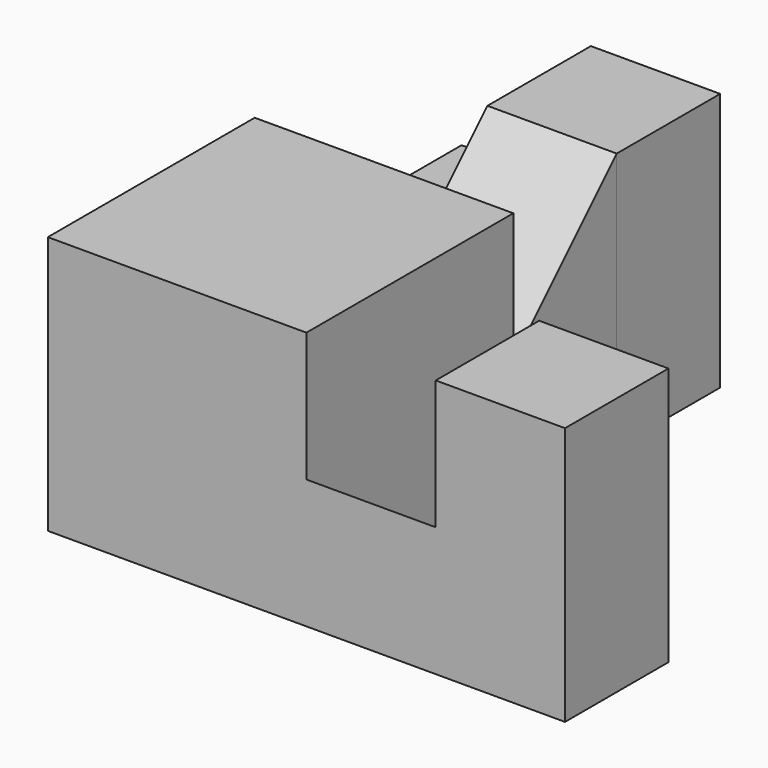
from build123d import *

# Parameters (mm, degrees)
F0_W     = 8
F0_H     = 8
F1_DEPTH = 16
F2_DEPTH = 8
F3_DEPTH = 16
F4_DEPTH = 8
F5_DEPTH = 16
F6_DEPTH = 16
F7_SIZE  = 7.99999
F8_SIZE  = 7.99999


# Not quite as in the source:
# - a fillet or chamfer is up to 0.001 mm smaller than in the source, because OpenCascade refuses the exact size


with BuildPart() as f1:
    # F0 (on Top) → F1 (new body)
    with BuildSketch(Plane.XY):
        with Locations((-2.9367977926, -12)):
            Rectangle(F0_W, F0_H)
    extrude(amount=F1_DEPTH)

    # F0 (on Top) → F2 (join)
    with BuildSketch(Plane.XY):
        with Locations((-10.9367977926, -12)):
            Rectangle(F0_W, F0_H)
    extrude(amount=F2_DEPTH)

    # F0 (on Top) → F3 (join)
    with BuildSketch(Plane.XY):
        Polygon((-22.9367977926, 0), (-30.9367977926, 0), (-30.9367977926, -16), (-14.9367977926, -16), (-14.9367977926, -8), (-14.9367977926, 0), align=None)
    extrude(amount=F3_DEPTH)

    # F0 (on Top) → F4 (join)
    with BuildSketch(Plane.XY):
        Polygon((-22.9367977926, 16), (-30.9367977926, 16), (-30.9367977926, 0), (-22.9367977926, 0), (-22.9367977926, 8), align=None)
    extrude(amount=F4_DEPTH)

    # F0 (on Top) → F5 (join)
    with BuildSketch(Plane.XY):
        with Locations((-18.9367977926, 12)):
            Rectangle(F0_W, F0_H)
    extrude(amount=F5_DEPTH)

    # F7 (size 8 in the source; OpenCascade refuses exactly that, so slightly less here)
    f7_edges = [f1.edges().sort_by_distance(p)[0] for p in [
        (-10.936798, -8, 8),
    ]]
    chamfer(f7_edges, length=F7_SIZE)


with BuildPart() as f6:
    # F0 (on Top) → F6 (new body)
    with BuildSketch(Plane.XY):
        with Locations((-18.9367977926, 4)):
            Rectangle(F0_W, F0_H)
    extrude(amount=F6_DEPTH)

    # F8 (size 8 in the source; OpenCascade refuses exactly that, so slightly less here)
    f8_edges = [f6.edges().sort_by_distance(p)[0] for p in [
        (-18.936798, 0, 16),
    ]]
    chamfer(f8_edges, length=F8_SIZE)


solid = Compound([f1.part, f6.part])
